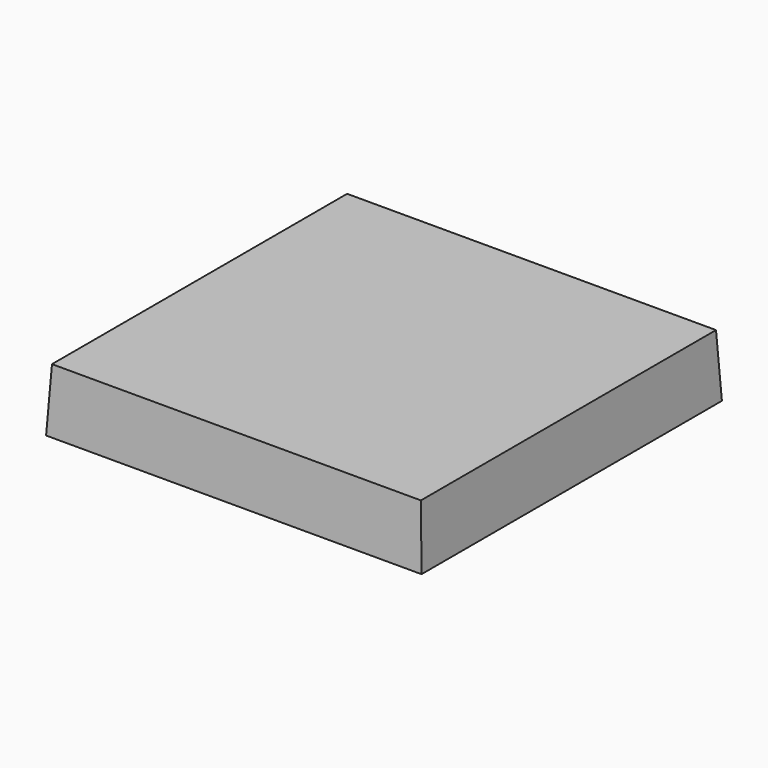
from build123d import *

# Parameters (mm, degrees)
F0_W     = 38.1
F0_H     = 38.1
F1_DEPTH = 6.35
F1_TAPER = 3


with BuildPart() as f1:
    # F0 (on Top) → F1 (new body)
    with BuildSketch(Plane.XY):
        Rectangle(F0_W, F0_H)
    extrude(amount=F1_DEPTH, taper=F1_TAPER)


solid = f1.part
